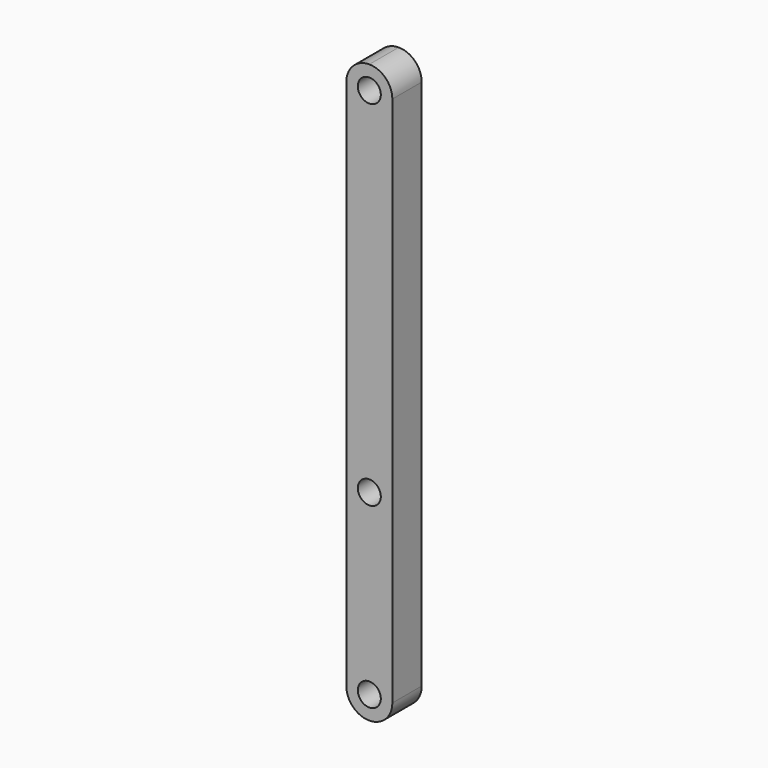
from build123d import *

# Parameters (mm, degrees)
F0_R     = 5.5
F1_DEPTH = 19.05
F2_DEPTH = 1.5


# Not quite as in the source:
# - a length typed as a fraction of an inch, garbled in the dataset ("3 / 203.2 mm" for 3/8 in), is restored
# - a feature names something its author has since deleted; it is built from what else it names


with BuildPart() as f1:
    # F0 (on Front) → F1 (new body)
    with BuildSketch(Plane.XZ):
        with BuildLine():
            Line((11, -127), (11, 127))
            ThreePointArc((11, 127), (7.7781745931, 134.7781745931), (0, 138))
            ThreePointArc((0, 138), (-7.7781745931, 134.7781745931), (-11, 127))
            Line((-11, 127), (-11, -127))
            ThreePointArc((-11, -127), (-7.7781745931, -134.7781745931), (0, -138))
            ThreePointArc((0, -138), (7.7781745931, -134.7781745931), (11, -127))
        make_face()
        with Locations((0, -127)):
            Circle(F0_R, mode=Mode.SUBTRACT)
        with Locations((0, -41.9999994338)):
            Circle(F0_R, mode=Mode.SUBTRACT)
        with Locations((0, 127)):
            Circle(F0_R, mode=Mode.SUBTRACT)
    extrude(amount=F1_DEPTH)

    # F0 (on Front) → F2 (cut)
    with BuildSketch(Plane.XZ):
        with BuildLine():
            Line((11, -127), (11, 127))
            ThreePointArc((11, 127), (7.7781745931, 134.7781745931), (0, 138))
            ThreePointArc((0, 138), (-7.7781745931, 134.7781745931), (-11, 127))
            Line((-11, 127), (-11, -127))
            ThreePointArc((-11, -127), (-7.7781745931, -134.7781745931), (0, -138))
            ThreePointArc((0, -138), (7.7781745931, -134.7781745931), (11, -127))
        make_face()
        with Locations((0, -127)):
            Circle(F0_R, mode=Mode.SUBTRACT)
        with Locations((0, -41.9999994338)):
            Circle(F0_R, mode=Mode.SUBTRACT)
        with Locations((0, 127)):
            Circle(F0_R, mode=Mode.SUBTRACT)
    extrude(amount=F2_DEPTH, mode=Mode.SUBTRACT)


solid = f1.part
